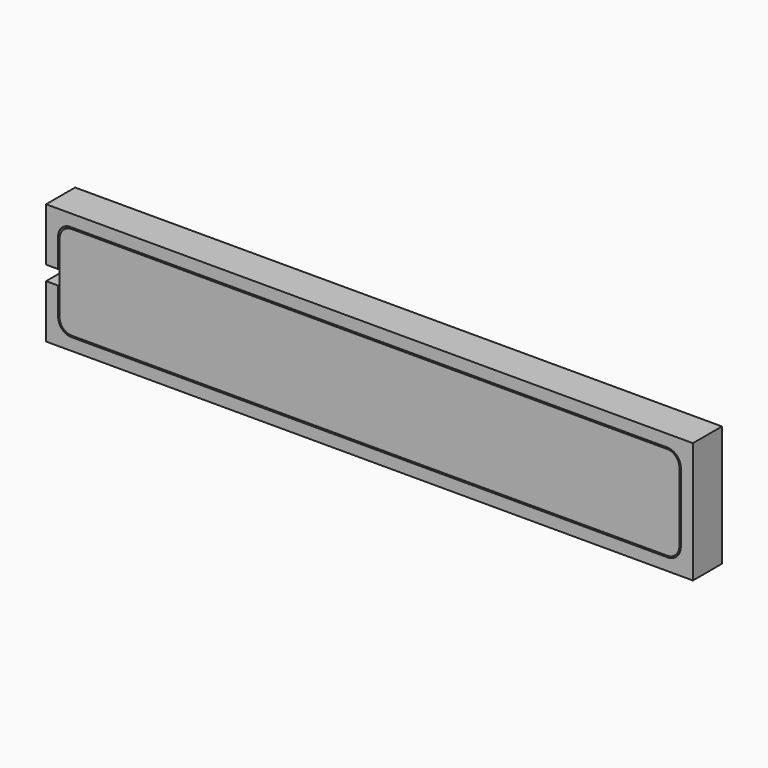
from build123d import *

# Parameters (mm, degrees)
F0_W     = 339.725
F0_H     = 63.5
F1_DEPTH = 19.05
F3_DEPTH = 12.7
F5_DEPTH = 8.89
F7_DEPTH = 7.62
F8_W     = 299.085
F8_H     = 16.002
F9_DEPTH = 25.4


with BuildPart() as f1:
    # F0 (on Front) → F1 (new body)
    with BuildSketch(Plane.XZ):
        with Locations((169.8625, 31.75)):
            Rectangle(F0_W, F0_H)
    extrude(amount=F1_DEPTH)

    # F2 (on face) → F3 (cut)
    with BuildSketch(Plane.XZ.offset(19.05)):
        with BuildLine():
            Line((313.563, 44.45), (13.462, 44.45))
            ThreePointArc((13.462, 44.45), (8.4330565722, 42.3669434278), (6.35, 37.338))
            Line((6.35, 37.338), (6.35, 35.56))
            Line((6.35, 35.56), (0, 35.56))
            Line((0, 35.56), (0, 27.94))
            Line((0, 27.94), (6.35, 27.94))
            Line((6.35, 27.94), (6.35, 26.162))
            ThreePointArc((6.35, 26.162), (8.4330565722, 21.1330565722), (13.462, 19.05))
            Line((13.462, 19.05), (313.563, 19.05))
            ThreePointArc((313.563, 19.05), (318.5919434278, 21.1330565722), (320.675, 26.162))
            Line((320.675, 26.162), (320.675, 37.338))
            ThreePointArc((320.675, 37.338), (318.5919434278, 42.3669434278), (313.563, 44.45))
        make_face()
    extrude(amount=-F3_DEPTH, mode=Mode.SUBTRACT)

    # F4 (on face) → F5 (cut)
    with BuildSketch(Plane.XZ.offset(19.05)):
        with BuildLine():
            Line((326.263, 57.15), (12.7, 57.15))
            ThreePointArc((12.7, 57.15), (8.2098719395, 55.2901280605), (6.35, 50.8))
            Line((6.35, 50.8), (6.35, 37.338))
            ThreePointArc((6.35, 37.338), (8.4330565722, 42.3669434278), (13.462, 44.45))
            Line((13.462, 44.45), (313.563, 44.45))
            ThreePointArc((313.563, 44.45), (318.5919434278, 42.3669434278), (320.675, 37.338))
            Line((320.675, 37.338), (320.675, 26.162))
            ThreePointArc((320.675, 26.162), (318.5919434278, 21.1330565722), (313.563, 19.05))
            Line((313.563, 19.05), (13.462, 19.05))
            ThreePointArc((13.462, 19.05), (8.4330565722, 21.1330565722), (6.35, 26.162))
            Line((6.35, 26.162), (6.35, 13.462))
            ThreePointArc((6.35, 13.462), (8.4330565722, 8.4330565722), (13.462, 6.35))
            Line((13.462, 6.35), (326.263, 6.35))
            ThreePointArc((326.263, 6.35), (331.2919434278, 8.4330565722), (333.375, 13.462))
            Line((333.375, 13.462), (333.375, 50.038))
            ThreePointArc((333.375, 50.038), (331.2919434278, 55.0669434278), (326.263, 57.15))
        make_face()
    extrude(amount=-F5_DEPTH, mode=Mode.SUBTRACT)

    # F8 (on face) → F9 (cut)
    with BuildSketch(Plane(origin=(0, 0, 0), x_dir=(-1, 0, 0), z_dir=(0, 1, 0))):
        with Locations((-169.8625, 31.75)):
            Rectangle(F8_W, F8_H)
    extrude(amount=-F9_DEPTH, mode=Mode.SUBTRACT)


with BuildPart() as f7:
    # F6 (on face) → F7 (new body)
    with BuildSketch(Plane.XZ.offset(19.05)):
        with BuildLine():
            Line((326.263, 56.388), (13.462, 56.388))
            ThreePointArc((13.462, 56.388), (8.9718719395, 54.5281280605), (7.112, 50.038))
            Line((7.112, 50.038), (7.112, 13.462))
            ThreePointArc((7.112, 13.462), (8.9718719395, 8.9718719395), (13.462, 7.112))
            Line((13.462, 7.112), (326.263, 7.112))
            ThreePointArc((326.263, 7.112), (330.7531280605, 8.9718719395), (332.613, 13.462))
            Line((332.613, 13.462), (332.613, 50.038))
            ThreePointArc((332.613, 50.038), (330.7531280605, 54.5281280605), (326.263, 56.388))
        make_face()
    extrude(amount=-F7_DEPTH)


solid = Compound([f1.part, f7.part])
